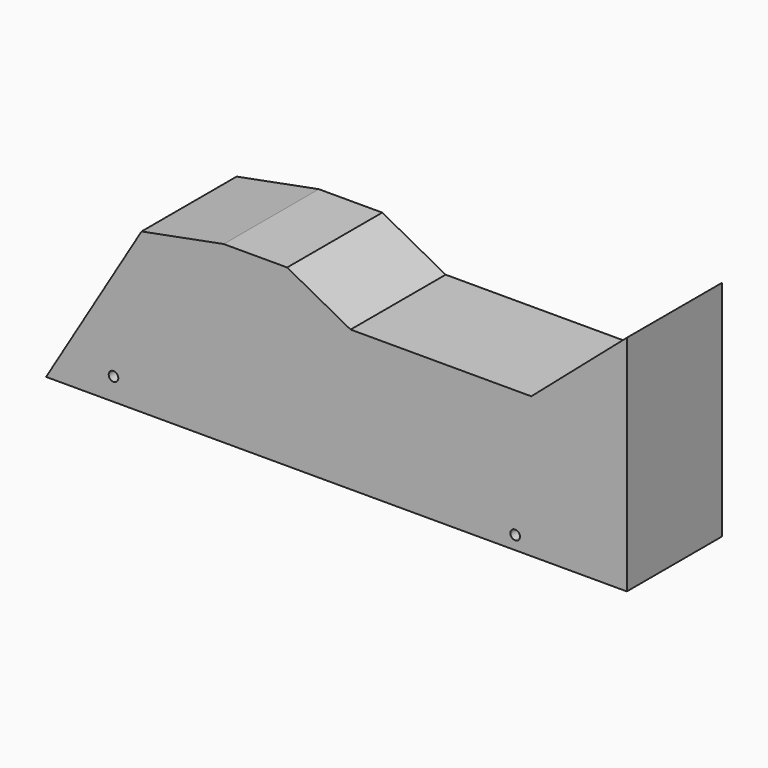
from build123d import *

# Parameters (mm, degrees)
F0_R     = 1.075
F1_DEPTH = 26.6
F2_DEPTH = 158
F4_DEPTH = 26.601


# Not quite as in the source:
# - an extrude ends at something that could not be found from the text; its depth is read off the source's solid


with BuildPart() as f1:
    # F0 (on Front) → F1 (new body)
    with BuildSketch(Plane.XZ):
        Polygon((50, 25), (-50, 25), (-80, -25), (-50, -25), (25, -25), (50, -25), align=None)
        with Locations((-64.9039745331, -20)):
            Circle(F0_R, mode=Mode.SUBTRACT)
        with Locations((25, -22)):
            Circle(F0_R, mode=Mode.SUBTRACT)
    extrude(amount=F1_DEPTH)

    # F0 (on Front) → F2 (cut, through all)
    with BuildSketch(Plane.XZ):
        with Locations((-64.9039745331, -20)):
            Circle(F0_R)
    extrude(amount=-F2_DEPTH, mode=Mode.SUBTRACT)

    # F3 (on face) → F4 (cut, through all)
    with BuildSketch(Plane(origin=(0, 0, 0), x_dir=(-1, 0, 0), z_dir=(0, 1, 0))):
        Polygon((50, 25), (-50, 25), (-28.6072827876, 6.4954175614), (11.8362475187, 6.4954175614), (26.036022231, 14.1141144559), (40.2304567397, 14.1141144559), (58.63198501, 10.6133583166), align=None)
    extrude(amount=-F4_DEPTH, mode=Mode.SUBTRACT)


solid = f1.part
